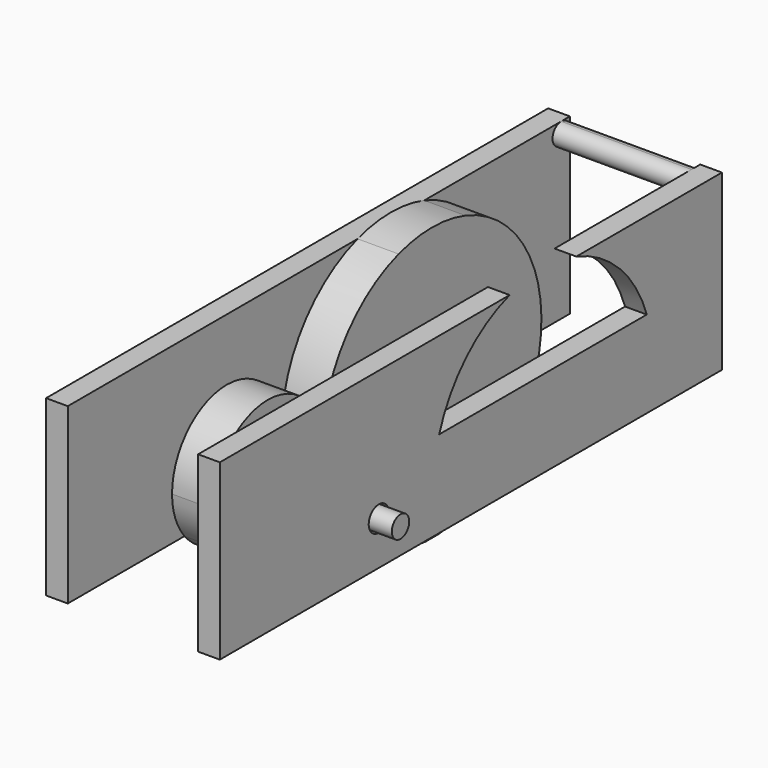
from build123d import *

# Parameters (mm, degrees)
F0_R      = 1.8415
F0_R_2    = 1.5875
F1_DEPTH  = 3.175
F2_DEPTH  = 19.05
F3_R      = 1.8415
F4_DEPTH  = 3.175
F3_R_2    = 1.5875
F5_DEPTH  = 3.175
F6_DEPTH  = 6
F7_DEPTH  = 6
F8_DEPTH  = 3.175
F9_DEPTH  = 25.4
F10_DEPTH = 6


# Not quite as in the source:
# - a feature names something its author has since deleted; it is built from what else it names


with BuildPart() as f1:
    # F0 (on Right) → F1 (new body)
    with BuildSketch(Plane.YZ):
        with BuildLine():
            Line((26.1329581332, 12.7), (29.4426713393, 12.7))
            ThreePointArc((29.4426713393, 12.7), (34.3624639947, 20.5882408837), (42.3170650669, 25.4))
            Line((42.3170650669, 25.4), (41.8216693056, 25.4))
            Line((41.8216693056, 25.4), (35.8211970083, 25.4))
            Line((35.8211970083, 25.4), (-10.6421632251, 25.4))
            Line((-10.6421632251, 25.4), (-10.6421632251, 0))
            Line((-10.6421632251, 0), (10.6827154167, 0))
            ThreePointArc((10.6827154167, 0), (12.0578367749, 14.0751213583), (26.1329581332, 12.7))
        make_face()
        with BuildLine():
            ThreePointArc((67.3730022106, 0), (68.1474328791, 3.1331155377), (68.4078367749, 6.35))
            ThreePointArc((68.4078367749, 6.35), (68.1474328791, 9.5668844623), (67.3730022106, 12.7))
            Line((67.3730022106, 12.7), (29.4426713393, 12.7))
            ThreePointArc((29.4426713393, 12.7), (28.6682406708, 9.5668844623), (28.4078367749, 6.35))
            ThreePointArc((28.4078367749, 6.35), (28.6682406708, 3.1331155377), (29.4426713393, 0))
            Line((29.4426713393, 0), (67.3730022106, 0))
        make_face()
        with Locations((48.4078367749, 6.35)):
            Circle(F0_R, mode=Mode.SUBTRACT)
        with BuildLine():
            ThreePointArc((54.498608483, 25.4), (62.4532095552, 20.5882408837), (67.3730022106, 12.7))
            Line((67.3730022106, 12.7), (74.2828367749, 12.7))
            Line((74.2828367749, 12.7), (74.2828367749, 0))
            Line((74.2828367749, 0), (80.2833090723, 0))
            Line((80.2833090723, 0), (81.1078367749, 0))
            Line((81.1078367749, 0), (81.1078367749, 23.8125))
            ThreePointArc((81.1078367749, 23.8125), (78.3978047598, 22.6899679849), (79.5203367749, 25.4))
            Line((79.5203367749, 25.4), (54.498608483, 25.4))
        make_face()
        with BuildLine():
            Line((22.0578367749, 12.7), (26.1329581332, 12.7))
            ThreePointArc((26.1329581332, 12.7), (12.0578367749, 14.0751213583), (10.6827154167, 0))
            Line((10.6827154167, 0), (22.0578367749, 0))
            Line((22.0578367749, 0), (22.0578367749, 12.7))
        make_face()
        with Locations((18.4078367749, 6.35)):
            Circle(F0_R, mode=Mode.SUBTRACT)
        with BuildLine():
            ThreePointArc((67.3730022106, 12.7), (68.1474328791, 9.5668844623), (68.4078367749, 6.35))
            ThreePointArc((68.4078367749, 6.35), (68.1474328791, 3.1331155377), (67.3730022106, 0))
            Line((67.3730022106, 0), (73.4878367749, 0))
            Line((73.4878367749, 0), (74.2828367749, 0))
            Line((74.2828367749, 0), (74.2828367749, 12.7))
            Line((74.2828367749, 12.7), (67.3730022106, 12.7))
        make_face()
        with BuildLine():
            ThreePointArc((26.1329581332, 0), (27.8219541946, 2.9774055671), (28.4078367749, 6.35))
            ThreePointArc((28.4078367749, 6.35), (27.8219541946, 9.7225944329), (26.1329581332, 12.7))
            Line((26.1329581332, 12.7), (22.0578367749, 12.7))
            Line((22.0578367749, 12.7), (22.0578367749, 0))
            Line((22.0578367749, 0), (26.1329581332, 0))
        make_face()
        with Locations((48.4078367749, 6.35)):
            Circle(F0_R)
        with Locations((48.4078367749, 6.35)):
            Circle(F0_R_2, mode=Mode.SUBTRACT)
        with Locations((48.4078367749, 6.35)):
            Circle(F0_R_2)
        with BuildLine():
            ThreePointArc((81.1078367749, 23.8125), (80.6428687901, 24.9350320151), (79.5203367749, 25.4))
            ThreePointArc((79.5203367749, 25.4), (78.3978047598, 22.6899679849), (81.1078367749, 23.8125))
        make_face()
        with BuildLine():
            ThreePointArc((28.4078367749, 6.35), (28.6682406708, 9.5668844623), (29.4426713393, 12.7))
            Line((29.4426713393, 12.7), (26.1329581332, 12.7))
            ThreePointArc((26.1329581332, 12.7), (27.8219541946, 9.7225944329), (28.4078367749, 6.35))
        make_face()
        with BuildLine():
            Line((26.1329581332, 0), (29.4426713393, 0))
            ThreePointArc((29.4426713393, 0), (28.6682406708, 3.1331155377), (28.4078367749, 6.35))
            ThreePointArc((28.4078367749, 6.35), (27.8219541946, 2.9774055671), (26.1329581332, 0))
        make_face()
        with BuildLine():
            Line((81.1078367749, 25.4), (79.5203367749, 25.4))
            ThreePointArc((79.5203367749, 25.4), (80.6428687901, 24.9350320151), (81.1078367749, 23.8125))
            Line((81.1078367749, 23.8125), (81.1078367749, 25.4))
        make_face()
    extrude(amount=F1_DEPTH)


with BuildPart() as f2:
    # F0 (on Right) → F2 (new body)
    with BuildSketch(Plane.YZ):
        with BuildLine():
            ThreePointArc((81.1078367749, 23.8125), (80.6428687901, 24.9350320151), (79.5203367749, 25.4))
            ThreePointArc((79.5203367749, 25.4), (78.3978047598, 22.6899679849), (81.1078367749, 23.8125))
        make_face()
    extrude(amount=-F2_DEPTH)


with BuildPart() as f4:
    # F3 (on face) → F4 (new body)
    with BuildSketch(Plane(origin=(-19.05, 0, 0), x_dir=(0, -1, 0), z_dir=(-1, 0, 0))):
        with BuildLine():
            Line((-79.5203367749, 25.4), (-81.1078367749, 25.4))
            Line((-81.1078367749, 25.4), (-81.1078367749, 23.8125))
            ThreePointArc((-81.1078367749, 23.8125), (-80.6428687901, 24.9350320151), (-79.5203367749, 25.4))
        make_face()
        with BuildLine():
            Line((-54.498608483, 25.4), (-79.5203367749, 25.4))
            ThreePointArc((-79.5203367749, 25.4), (-78.3978047598, 24.9350320151), (-77.9328367749, 23.8125))
            ThreePointArc((-77.9328367749, 23.8125), (-79.5203367749, 22.225), (-81.1078367749, 23.8125))
            Line((-81.1078367749, 23.8125), (-81.1078367749, 0))
            Line((-81.1078367749, 0), (-67.3730022106, 0))
            ThreePointArc((-67.3730022106, 0), (-66.2471191747, 15.3921238358), (-54.498608483, 25.4))
        make_face()
        with BuildLine():
            ThreePointArc((-77.9328367749, 23.8125), (-78.3978047598, 24.9350320151), (-79.5203367749, 25.4))
            ThreePointArc((-79.5203367749, 25.4), (-80.6428687901, 24.9350320151), (-81.1078367749, 23.8125))
            ThreePointArc((-81.1078367749, 23.8125), (-79.5203367749, 22.225), (-77.9328367749, 23.8125))
        make_face()
        with BuildLine():
            Line((-42.3170650669, 25.4), (-54.498608483, 25.4))
            ThreePointArc((-54.498608483, 25.4), (-66.2471191747, 15.3921238358), (-67.3730022106, 0))
            Line((-67.3730022106, 0), (-64.2828367749, 0))
            Line((-64.2828367749, 0), (-64.2828367749, 12.7))
            Line((-64.2828367749, 12.7), (-42.0578367749, 12.7))
            Line((-42.0578367749, 12.7), (-42.0578367749, 6.35))
            Line((-42.0578367749, 6.35), (-42.0578367749, 0))
            Line((-42.0578367749, 0), (-29.4426713393, 0))
            ThreePointArc((-29.4426713393, 0), (-28.6682406708, 3.1331155377), (-28.4078367749, 6.35))
            ThreePointArc((-28.4078367749, 6.35), (-32.2551986907, 18.1437391407), (-42.3170650669, 25.4))
        make_face()
        with BuildLine():
            Line((10.6421632251, 25.4), (-42.3170650669, 25.4))
            ThreePointArc((-42.3170650669, 25.4), (-32.2551986907, 18.1437391407), (-28.4078367749, 6.35))
            ThreePointArc((-28.4078367749, 6.35), (-18.4078367749, 16.35), (-8.4078367749, 6.35))
            ThreePointArc((-8.4078367749, 6.35), (-8.9937193553, 2.9774055671), (-10.6827154167, 0))
            Line((-10.6827154167, 0), (10.6421632251, 0))
            Line((10.6421632251, 0), (10.6421632251, 25.4))
        make_face()
        with BuildLine():
            ThreePointArc((-26.1329581332, 0), (-27.8219541946, 2.9774055671), (-28.4078367749, 6.35))
            ThreePointArc((-28.4078367749, 6.35), (-28.6682406708, 3.1331155377), (-29.4426713393, 0))
            Line((-29.4426713393, 0), (-26.1329581332, 0))
        make_face()
        with BuildLine():
            ThreePointArc((-8.4078367749, 6.35), (-18.4078367749, 16.35), (-28.4078367749, 6.35))
            ThreePointArc((-28.4078367749, 6.35), (-27.8219541946, 2.9774055671), (-26.1329581332, 0))
            Line((-26.1329581332, 0), (-10.6827154167, 0))
            ThreePointArc((-10.6827154167, 0), (-8.9937193553, 2.9774055671), (-8.4078367749, 6.35))
        make_face()
        with Locations((-18.4078367749, 6.35)):
            Circle(F3_R, mode=Mode.SUBTRACT)
    extrude(amount=F4_DEPTH)


with BuildPart() as f5:
    # F3 (on face) → F5 (new body)
    with BuildSketch(Plane(origin=(-19.05, 0, 0), x_dir=(0, -1, 0), z_dir=(-1, 0, 0))):
        with Locations((-48.4078367749, 6.35)):
            Circle(F3_R_2)
    extrude(amount=F5_DEPTH)

    # F3 (on face) → F6 (join)
    with BuildSketch(Plane(origin=(-19.05, 0, 0), x_dir=(0, -1, 0), z_dir=(-1, 0, 0))):
        with Locations((-48.4078367749, 6.35)):
            Circle(F3_R_2)
    extrude(amount=-F6_DEPTH)


with BuildPart() as f7:
    # F3 (on face) → F7 (new body)
    with BuildSketch(Plane(origin=(-19.05, 0, 0), x_dir=(0, -1, 0), z_dir=(-1, 0, 0))):
        with BuildLine():
            Line((-42.3170650669, 25.4), (-54.498608483, 25.4))
            ThreePointArc((-54.498608483, 25.4), (-66.2471191747, 15.3921238358), (-67.3730022106, 0))
            Line((-67.3730022106, 0), (-64.2828367749, 0))
            Line((-64.2828367749, 0), (-64.2828367749, 12.7))
            Line((-64.2828367749, 12.7), (-42.0578367749, 12.7))
            Line((-42.0578367749, 12.7), (-42.0578367749, 6.35))
            Line((-42.0578367749, 6.35), (-42.0578367749, 0))
            Line((-42.0578367749, 0), (-29.4426713393, 0))
            ThreePointArc((-29.4426713393, 0), (-28.6682406708, 3.1331155377), (-28.4078367749, 6.35))
            ThreePointArc((-28.4078367749, 6.35), (-32.2551986907, 18.1437391407), (-42.3170650669, 25.4))
        make_face()
        with BuildLine():
            Line((-64.2828367749, 0), (-67.3730022106, 0))
            ThreePointArc((-67.3730022106, 0), (-48.4078367749, -13.65), (-29.4426713393, 0))
            Line((-29.4426713393, 0), (-42.0578367749, 0))
            Line((-42.0578367749, 0), (-64.2828367749, 0))
        make_face()
        Polygon((-64.2828367749, 12.7), (-64.2828367749, 0), (-42.0578367749, 0), (-42.0578367749, 6.35), (-42.0578367749, 12.7), align=None)
        with Locations((-48.4078367749, 6.35)):
            Circle(F3_R, mode=Mode.SUBTRACT)
        with Locations((-48.4078367749, 6.35)):
            Circle(F3_R)
        with Locations((-48.4078367749, 6.35)):
            Circle(F3_R_2, mode=Mode.SUBTRACT)
        with BuildLine():
            ThreePointArc((-42.3170650669, 25.4), (-48.4078367749, 26.35), (-54.498608483, 25.4))
            Line((-54.498608483, 25.4), (-42.3170650669, 25.4))
        make_face()
    extrude(amount=-F7_DEPTH)


with BuildPart() as f8:
    # F3 (on face) → F8 (new body)
    with BuildSketch(Plane(origin=(-19.05, 0, 0), x_dir=(0, -1, 0), z_dir=(-1, 0, 0))):
        with Locations((-18.4078367749, 6.35)):
            Circle(F3_R_2)
    extrude(amount=F8_DEPTH)

    # F3 (on face) → F9 (join)
    with BuildSketch(Plane(origin=(-19.05, 0, 0), x_dir=(0, -1, 0), z_dir=(-1, 0, 0))):
        with Locations((-18.4078367749, 6.35)):
            Circle(F3_R_2)
    extrude(amount=-F9_DEPTH)


with BuildPart() as f10:
    # F3 (on face) → F10 (new body)
    with BuildSketch(Plane(origin=(-19.05, 0, 0), x_dir=(0, -1, 0), z_dir=(-1, 0, 0))):
        with BuildLine():
            ThreePointArc((-8.4078367749, 6.35), (-18.4078367749, 16.35), (-28.4078367749, 6.35))
            ThreePointArc((-28.4078367749, 6.35), (-27.8219541946, 2.9774055671), (-26.1329581332, 0))
            Line((-26.1329581332, 0), (-10.6827154167, 0))
            ThreePointArc((-10.6827154167, 0), (-8.9937193553, 2.9774055671), (-8.4078367749, 6.35))
        make_face()
        with Locations((-18.4078367749, 6.35)):
            Circle(F3_R, mode=Mode.SUBTRACT)
        with Locations((-18.4078367749, 6.35)):
            Circle(F3_R)
        with Locations((-18.4078367749, 6.35)):
            Circle(F3_R_2, mode=Mode.SUBTRACT)
        with BuildLine():
            Line((-10.6827154167, 0), (-26.1329581332, 0))
            ThreePointArc((-26.1329581332, 0), (-18.4078367749, -3.65), (-10.6827154167, 0))
        make_face()
    extrude(amount=-F10_DEPTH)


solid = Compound([f1.part, f2.part, f4.part, f5.part, f7.part, f8.part, f10.part])
